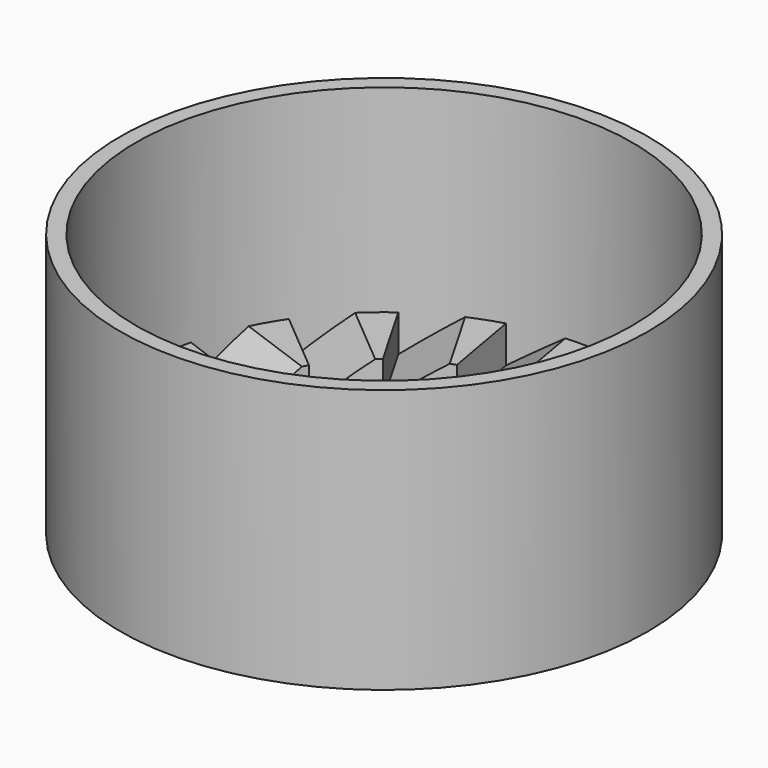
from build123d import *

# Parameters (mm, degrees)
F0_R            = 20
F1_DEPTH        = 20
F2_R            = 18.8
F3_DEPTH        = 15
F4_R            = 12.8
F5_DEPTH        = 25
F7_END_RADIUS   = 18.8
F7_REACH        = 24.884098355
F7_COPIES_COUNT = 18


# Not quite as in the source:
# - a pattern or mirror of a feature is missing from the dataset's text; its kind, count and spacing are read off the source's solid


with BuildPart() as f1:
    # F0 (on Top) → F1 (new body)
    with BuildSketch(Plane.XY):
        Circle(F0_R)
    extrude(amount=F1_DEPTH)

    # F2 (on face) → F3 (cut)
    with BuildSketch(Plane.XY.offset(20)):
        Circle(F2_R)
    extrude(amount=-F3_DEPTH, mode=Mode.SUBTRACT)

    # F4 (on face) → F5 (cut)
    with BuildSketch(Plane.XY.offset(5)):
        Circle(F4_R)
    extrude(amount=-F5_DEPTH, mode=Mode.SUBTRACT)

    f7_end = (Plane.XY.offset(12.5) * Cylinder(F7_END_RADIUS, 169.7681967101, mode=Mode.PRIVATE)).faces().sort_by_distance((-18.8, 0, 12.5))[0]
    # F6 (on Right) → F7 (cut, up to the whole of a round face its end follows)
    with BuildSketch(Plane.YZ):
        Polygon((-2, 5), (-2, 2.1991698472), (0, 3.5995849236), (2, 5), align=None)
    f7_long = extrude(amount=-F7_REACH, mode=Mode.PRIVATE)
    f7 = split(f7_long, bisect_by=f7_end, keep=Keep.BOTTOM, mode=Mode.PRIVATE)
    add(f7, mode=Mode.SUBTRACT)

    # F7_copies: F7 ×18 about axis
    f7_copies_axis = Axis((0, 0, 0), (0, 0, 1))
    for i in range(1, F7_COPIES_COUNT):
        add(f7.rotate(f7_copies_axis, i * 360 / F7_COPIES_COUNT), mode=Mode.SUBTRACT)


solid = f1.part
